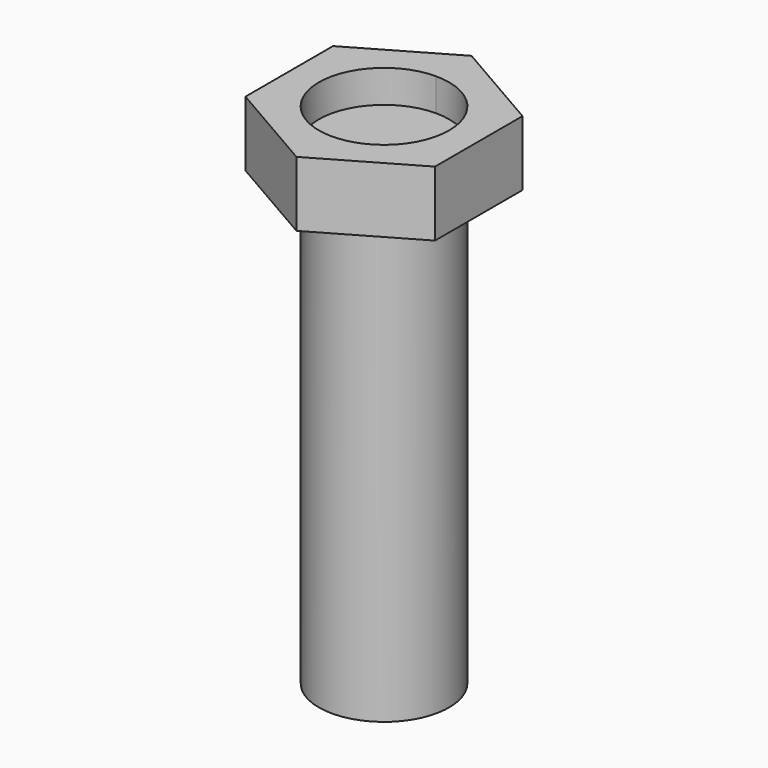
from build123d import *

# Parameters (mm, degrees)
F0_W     = 1
F0_H     = 6.8
F3_DEPTH = 1
F4_R     = 1
F5_DEPTH = 0.5


# Not quite as in the source:
# - a pattern or mirror of a feature is missing from the dataset's text; its kind, count and spacing are read off the source's solid


with BuildPart() as f1:
    # F0 (on Front) → F1 (revolve)
    with BuildSketch(Plane.XZ):
        with Locations((-0.5, 3.4)):
            Rectangle(F0_W, F0_H)
    revolve(axis=Axis((0, 0, 3.4), (0, 0, 1)))

    # F1_copies: F1 across plane


with BuildPart() as f1_1:
    add(f1.part)
    add(f1.part.mirror(Plane.XY.offset(3.65)))

    # F2 (on face) → F3 (join)
    with BuildSketch(Plane.XY.offset(6.8)):
        Polygon((1.4549226784, 0.84), (0, 1.68), (-1.4549226784, 0.84), (-1.4549226784, -0.84), (0, -1.68), (1.4549226784, -0.84), align=None)
        with BuildLine():
            ThreePointArc((1, 0), (-0.7071067812, -0.7071067812), (0, 1))
            ThreePointArc((0, 1), (0.7071067812, 0.7071067812), (1, 0))
        make_face(mode=Mode.SUBTRACT)
    extrude(amount=F3_DEPTH)

    # F4 (on face) → F5 (cut)
    with BuildSketch(Plane.XY.offset(7.8)):
        Circle(F4_R)
    extrude(amount=-F5_DEPTH, mode=Mode.SUBTRACT)


solid = f1_1.part
